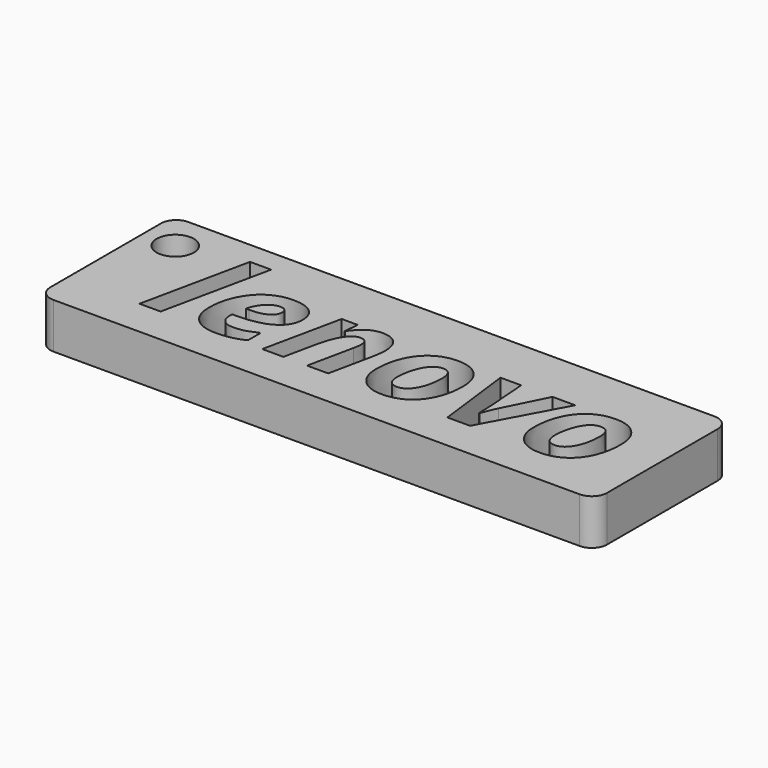
from build123d import *

# Parameters (mm, degrees)
F0_R         = 6.1345408447
F1_DEPTH     = 15
F3_TEXT_SIZE = 47.3529456132
F4_DEPTH     = 10


# Not quite as in the source:
# - Text() gives the source's letters only with a copy of the font that has no kerning and outlines rounded to 1/6400 em; it was checked with that copy


with BuildPart() as f1:
    # F0 (on Top) → F1 (new body)
    with BuildSketch(Plane.XY):
        with BuildLine():
            Line((86.0362228751, 49.9367676675), (-87.404961586, 49.9367676675))
            ThreePointArc((-87.404961586, 49.9367676675), (-90.9404954919, 48.4723015735), (-92.404961586, 44.9367676675))
            Line((-92.404961586, 44.9367676675), (-92.404961586, -0.6514707394))
            ThreePointArc((-92.404961586, -0.6514707394), (-90.9404954919, -4.1870046453), (-87.404961586, -5.6514707394))
            Line((-87.404961586, -5.6514707394), (86.0362228751, -5.6514707394))
            ThreePointArc((86.0362228751, -5.6514707394), (89.5717567811, -4.1870046453), (91.0362228751, -0.6514707394))
            Line((91.0362228751, -0.6514707394), (91.0362228751, 44.9367676675))
            ThreePointArc((91.0362228751, 44.9367676675), (89.5717567811, 48.4723015735), (86.0362228751, 49.9367676675))
        make_face()
        with Locations((-81.7756205797, 37.5333428383)):
            Circle(F0_R, mode=Mode.SUBTRACT)
    extrude(amount=F1_DEPTH)

    # F3 (on offset) → F4 (cut)
    with BuildSketch(Plane.XY.offset(15)):
        with Locations((-69.6141654626, 6.5303887241)):
            Text('lenovo', F3_TEXT_SIZE, font='Open Sans', font_style=FontStyle.BOLDITALIC, text_align=(TextAlign.LEFT, TextAlign.BOTTOM))
    extrude(amount=-F4_DEPTH, mode=Mode.SUBTRACT)


solid = f1.part
